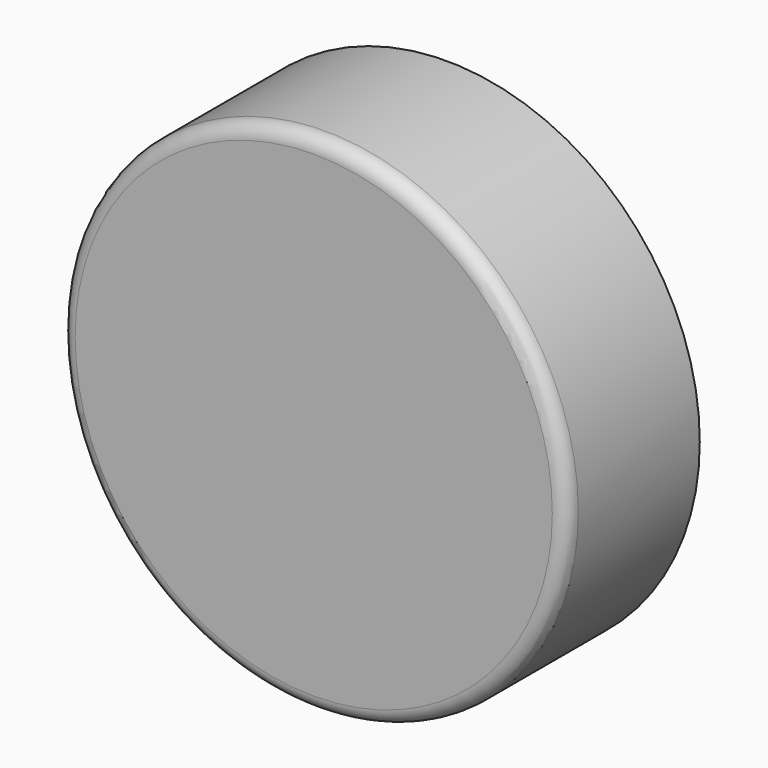
from build123d import *

# Parameters (mm, degrees)
F0_R     = 35
F1_DEPTH = 23
F2_T     = -1
F3_R     = 2


# Not quite as in the source:
# - a feature of the source that left no trace in its solid (it failed there, or was rolled back) is left out


with BuildPart() as f1:
    # F0 (on Front) → F1 (new body)
    with BuildSketch(Plane.XZ):
        Circle(F0_R)
    extrude(amount=F1_DEPTH)

    # F2
    f2_openings = [f1.faces().sort_by_distance(p)[0] for p in [
        (0, 0, 0),
    ]]
    offset(amount=F2_T, openings=f2_openings)

    # F3
    f3_edges = [f1.edges().sort_by_distance(p)[0] for p in [
        (-35, -23, 0),
    ]]
    fillet(f3_edges, radius=F3_R)


solid = f1.part
